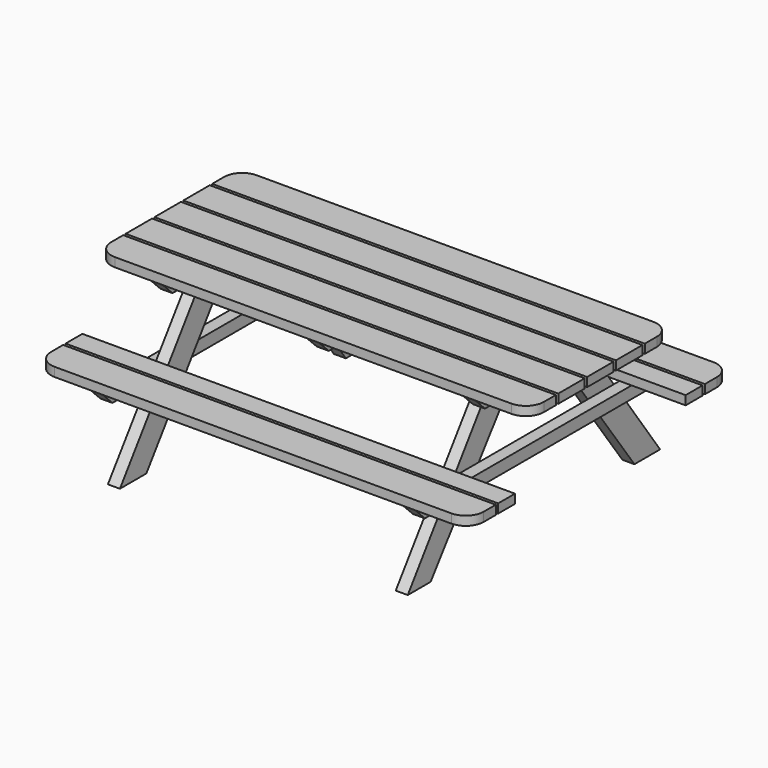
from build123d import *

# Parameters (mm, degrees)
F3_W       = 1828.8
F3_H       = 139.7
F4_DEPTH   = 38.1
F2_W       = 1828.8
F2_H       = 139.7
F5_R       = 76.2
F5_2_R     = 76.2
F6_W       = 1828.8
F6_H       = 88.9
F7_DEPTH   = 38.1
F6_H_2     = 139.7
F8_R       = 76.2
F8_2_R     = 76.2
F9_W       = 50.8
F9_H       = 749.3
F10_DEPTH  = 50.8
F12_SIZE   = 50.79999
F12_2_SIZE = 50.79999
F12_3_SIZE = 50.79999
F11_W      = 50.8
F11_H      = 1384.3
F13_DEPTH  = 50.8
F14_SIZE   = 50.79999
F14_2_SIZE = 50.79999
F15_W      = 50.8
F15_H      = 139.7
F16_W      = 50.8
F16_H      = 135.6702318695
F15_W_2    = 50.5662006634
F16_H_2    = 139.7
F16_H_3    = 120.8942294282


# Not quite as in the source:
# - a fillet or chamfer is up to 0.001 mm smaller than in the source, because OpenCascade refuses the exact size


with BuildPart() as f4:
    # F3 (on offset) → F4 (new body)
    with BuildSketch(Plane.XY.offset(622.3)):
        with Locations((0, 304.8)):
            Rectangle(F3_W, F3_H)
    extrude(amount=F4_DEPTH)

    # F5#2
    f5_2_edges = [f4.edges().sort_by_distance(p)[0] for p in [
        (914.4, 374.65, 641.35),
        (-914.4, 374.65, 641.35),
    ]]
    fillet(f5_2_edges, radius=F5_2_R)


with BuildPart() as f4b:
    # F3 (on offset) → F4, piece 2 (new body)
    with BuildSketch(Plane.XY.offset(622.3)):
        with Locations((0, 152.4)):
            Rectangle(F3_W, F3_H)
    extrude(amount=F4_DEPTH)

    # F15 (on offset) → F17 section 0
    with BuildSketch(Plane.XY.offset(622.3)):
        with Locations((608.33, 151.4005087376)):
            Rectangle(F15_W, F15_H)
    # F16 (on Top) → F17 section 1
    with BuildSketch(Plane.XY):
        with Locations((608.33, 598.9148840653)):
            Rectangle(F16_W, F16_H)
    loft()

    # F15 (on offset) → F18 section 0
    with BuildSketch(Plane.XY.offset(622.3)):
        with Locations((-608.4468996683, 151.3350016614)):
            Rectangle(F15_W_2, F15_H)
    # F16 (on Top) → F18 section 1
    with BuildSketch(Plane.XY):
        with Locations((-608.33, 596.9)):
            Rectangle(F16_W, F16_H_2)
    loft()


with BuildPart() as f4c:
    # F3 (on offset) → F4, piece 3 (new body)
    with BuildSketch(Plane.XY.offset(622.3)):
        with Locations((0, -152.4)):
            Rectangle(F3_W, F3_H)
    extrude(amount=F4_DEPTH)

    # F15 (on offset) → F19 section 0
    with BuildSketch(Plane.XY.offset(622.3)):
        with Locations((608.33, -153.4392811298)):
            Rectangle(F15_W, F15_H)
    # F16 (on Top) → F19 section 1
    with BuildSketch(Plane.XY):
        with Locations((608.33, -606.3028852859)):
            Rectangle(F16_W, F16_H_3)
    loft()

    # F15 (on offset) → F20 section 0
    with BuildSketch(Plane.XY.offset(622.3)):
        with Locations((-608.4468996683, -152.4910742103)):
            Rectangle(F15_W_2, F15_H)
    # F16 (on Top) → F20 section 1
    with BuildSketch(Plane.XY):
        with Locations((-608.33, -596.9)):
            Rectangle(F16_W, F16_H_2)
    loft()


with BuildPart() as f4d:
    # F3 (on offset) → F4, piece 4 (new body)
    with BuildSketch(Plane.XY.offset(622.3)):
        with Locations((0, -304.8)):
            Rectangle(F3_W, F3_H)
    extrude(amount=F4_DEPTH)

    # F5
    f5_edges = [f4d.edges().sort_by_distance(p)[0] for p in [
        (914.4, -374.65, 641.35),
        (-914.4, -374.65, 641.35),
    ]]
    fillet(f5_edges, radius=F5_R)


with BuildPart() as f4e:
    # F2 (on offset) → F4, piece 5 (new body)
    with BuildSketch(Plane.XY.offset(622.3)):
        Rectangle(F2_W, F2_H)
    extrude(amount=F4_DEPTH)


with BuildPart() as f7:
    # F6 (on offset) → F7 (new body)
    with BuildSketch(Plane.XY.offset(342.9)):
        with Locations((0, 495.3)):
            Rectangle(F6_W, F6_H)
    extrude(amount=F7_DEPTH)


with BuildPart() as f7b:
    # F6 (on offset) → F7, piece 2 (new body)
    with BuildSketch(Plane.XY.offset(342.9)):
        with Locations((0, -495.3)):
            Rectangle(F6_W, F6_H)
    extrude(amount=F7_DEPTH)


with BuildPart() as f7c:
    # F6 (on offset) → F7, piece 3 (new body)
    with BuildSketch(Plane.XY.offset(342.9)):
        with Locations((0, 622.3)):
            Rectangle(F6_W, F6_H_2)
    extrude(amount=F7_DEPTH)

    # F8#2
    f8_2_edges = [f7c.edges().sort_by_distance(p)[0] for p in [
        (-914.4, 692.15, 361.95),
        (914.4, 692.15, 361.95),
    ]]
    fillet(f8_2_edges, radius=F8_2_R)


with BuildPart() as f7d:
    # F6 (on offset) → F7, piece 4 (new body)
    with BuildSketch(Plane.XY.offset(342.9)):
        with Locations((0, -622.3)):
            Rectangle(F6_W, F6_H_2)
    extrude(amount=F7_DEPTH)

    # F8
    f8_edges = [f7d.edges().sort_by_distance(p)[0] for p in [
        (-914.4, -692.15, 361.95),
        (914.4, -692.15, 361.95),
    ]]
    fillet(f8_edges, radius=F8_R)


with BuildPart() as f10:
    # F9 (on offset) → F10 (new body)
    with BuildSketch(Plane.XY.offset(622.3)):
        with Locations((-660.4, 0)):
            Rectangle(F9_W, F9_H)
    extrude(amount=-F10_DEPTH)

    # F12 (size 50.8 in the source; OpenCascade refuses exactly that, so slightly less here)
    f12_edges = [f10.edges().sort_by_distance(p)[0] for p in [
        (-660.4, -374.65, 571.5),
        (-660.4, 374.65, 571.5),
    ]]
    chamfer(f12_edges, length=F12_SIZE)


with BuildPart() as f10b:
    # F9 (on offset) → F10, piece 2 (new body)
    with BuildSketch(Plane.XY.offset(622.3)):
        with Locations((660.4, 0)):
            Rectangle(F9_W, F9_H)
    extrude(amount=-F10_DEPTH)

    # F12#3 (size 50.8 in the source; OpenCascade refuses exactly that, so slightly less here)
    f12_3_edges = [f10b.edges().sort_by_distance(p)[0] for p in [
        (660.4, -374.65, 571.5),
        (660.4, 374.65, 571.5),
    ]]
    chamfer(f12_3_edges, length=F12_3_SIZE)


with BuildPart() as f10c:
    # F9 (on offset) → F10, piece 3 (new body)
    with BuildSketch(Plane.XY.offset(622.3)):
        Rectangle(F9_W, F9_H)
    extrude(amount=-F10_DEPTH)

    # F12#2 (size 50.8 in the source; OpenCascade refuses exactly that, so slightly less here)
    f12_2_edges = [f10c.edges().sort_by_distance(p)[0] for p in [
        (0, -374.65, 571.5),
        (0, 374.65, 571.5),
    ]]
    chamfer(f12_2_edges, length=F12_2_SIZE)


with BuildPart() as f13:
    # F11 (on offset) → F13 (new body)
    with BuildSketch(Plane.XY.offset(342.9)):
        with Locations((-660.4, 0)):
            Rectangle(F11_W, F11_H)
    extrude(amount=-F13_DEPTH)

    # F14 (size 50.8 in the source; OpenCascade refuses exactly that, so slightly less here)
    f14_edges = [f13.edges().sort_by_distance(p)[0] for p in [
        (-660.4, -692.15, 292.1),
        (-660.4, 692.15, 292.1),
    ]]
    chamfer(f14_edges, length=F14_SIZE)


with BuildPart() as f13b:
    # F11 (on offset) → F13, piece 2 (new body)
    with BuildSketch(Plane.XY.offset(342.9)):
        with Locations((660.4, 0)):
            Rectangle(F11_W, F11_H)
    extrude(amount=-F13_DEPTH)

    # F14#2 (size 50.8 in the source; OpenCascade refuses exactly that, so slightly less here)
    f14_2_edges = [f13b.edges().sort_by_distance(p)[0] for p in [
        (660.4, -692.15, 292.1),
        (660.4, 692.15, 292.1),
    ]]
    chamfer(f14_2_edges, length=F14_2_SIZE)


solid = Compound([f4.part, f4b.part, f4c.part, f4d.part, f4e.part, f7.part, f7b.part, f7c.part, f7d.part, f10.part, f10b.part, f10c.part, f13.part, f13b.part])
